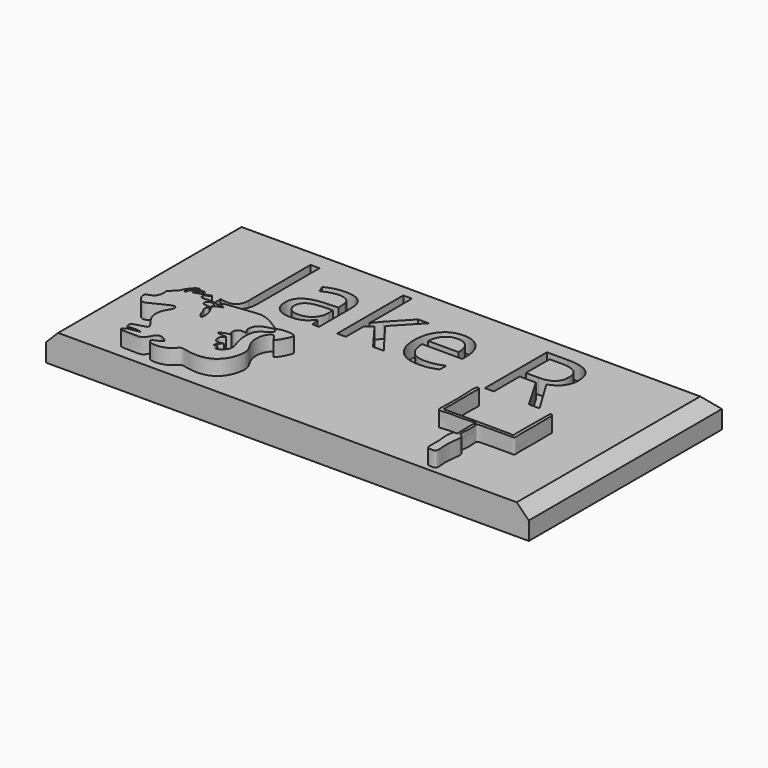
from build123d import *

# Parameters (mm, degrees)
F0_W         = 101.6
F0_H         = 50.8
F1_DEPTH     = 6.35
F2_TEXT_SIZE = 22.889892312
F3_DEPTH     = 3.175
F6_DEPTH     = 3.175
F8_DEPTH     = 3.175
F9_SIZE      = 2.54


# Not quite as in the source:
# - Text() gives the source's letters only with a copy of the font that has no kerning and outlines rounded to 1/6400 em; it was checked with that copy


with BuildPart() as f1:
    # F0 (on Top) → F1 (new body)
    with BuildSketch(Plane.XY):
        with Locations((31.7524990533, -6.3369355765)):
            Rectangle(F0_W, F0_H)
    extrude(amount=F1_DEPTH)

    # F2 (on face) → F3 (cut)
    with BuildSketch(Plane.XY.offset(6.35)):
        with Locations((-1.3590687886, -3.2846634276)):
            Text('Jake R', F2_TEXT_SIZE, font='Open Sans', text_align=(TextAlign.LEFT, TextAlign.BOTTOM))
    extrude(amount=-F3_DEPTH, mode=Mode.SUBTRACT)

    # F5 (on face) → F6 (join)
    with BuildSketch(Plane.XY.offset(6.35)):
        with BuildLine():
            add(Edge.make_bspline(
                [(-9.9473167211, -16.8291665614), (-9.6318161308, -16.6093979481), (-8.0839962394, -16.4614298786), (-7.9211876919, -14.0293243028), (-8.3789792586, -13.9112234461), (-6.3385914042, -12.0992000222), (-6.5202812577, -11.8356315571), (-5.2656681133, -10.0118497624), (-4.5534071308, -9.7378645456), (-4.2294561968, -9.7019648093), (-4.3980035932, -9.988698615), (-5.3176847151, -10.4409761465), (-5.7133396144, -11.440009908), (-5.7601749231, -12.0507048992), (-5.3250122812, -12.0166586319), (-5.5151695466, -11.2267993409), (-4.4172648305, -10.4678783041), (-3.8013369692, -10.2413822662), (-3.1664584015, -9.9795622858), (-2.9351873262, -10.0870364506), (-3.6173853606, -10.4333631624), (-4.4106140277, -10.9661153724), (-4.6578929311, -11.6389382333), (-2.9685088968, -10.872611876), (-1.7672060238, -10.5575074617), (-1.1369119673, -10.3099300849), (-1.3782200505, -10.7224404484), (-2.4536131421, -11.0524062418), (-2.3627095497, -12.0366415406), (-1.1805119076, -11.9653257133), (0.5407672641, -11.8701370936), (0.7217330171, -12.3150559399), (-0.4018086187, -12.270141763), (-0.8940503935, -13.3290837491), (-0.0457538349, -13.7435809238), (1.1398694142, -13.5461403967), (0.7699728306, -14.1837469378), (0.5285162187, -14.8135221399), (0.9767861849, -15.3013890012), (1.2067508203, -16.0261665589), (1.4266113794, -16.8041541097), (1.8335409915, -17.2417675619), (2.2896541555, -17.5865197382), (2.3269041493, -16.1396203305), (2.0902824393, -15.2175440987), (1.6059851597, -14.253562876), (1.3203956773, -13.6380943063), (0.8656034334, -13.378915598), (1.6536734035, -13.0102058821), (2.1442638998, -12.6770885728), (3.3244491956, -12.4108420977), (0.1829963842, -11.4779566095), (6.6402986528, -10.9518911639), (9.2079636257, -10.4311276641), (11.5736832476, -11.238028674), (13.213297199, -12.3934022949), (14.5980573697, -13.1660552716), (12.8123999886, -13.4588177694), (10.931038794, -14.193343875), (10.5901748999, -16.3206207186), (11.8353188414, -17.3818853519), (9.5427126702, -16.7472257612), (9.1994806574, -18.7963337624), (10.2773541237, -19.2600223908), (9.2663295553, -19.1819954863), (6.4967182387, -20.3558888921), (10.5627454218, -20.212945517), (8.8804020018, -20.8702686445), (8.9543814012, -21.9589086267), (9.3820569376, -22.9183607691), (11.461742552, -22.2172179196), (10.2513099098, -22.9519144726), (9.6568200022, -24.2677990338), (11.0083795729, -23.4196006133), (10.6327982369, -25.2961685937), (13.026023199, -23.6602826242), (12.8739516315, -21.9171844349), (11.9206539994, -19.6132841054), (11.888703896, -15.6842303702), (14.1445273132, -14.8208379496), (15.0950637719, -13.723427814), (13.9986766358, -13.2344335713), (15.4668397437, -12.5034113795), (18.2212563844, -12.7012871068), (18.3108018209, -13.7225720098), (16.5749799152, -16.8913138268), (16.2288416461, -15.7403926522), (15.1350726404, -14.4041878251), (13.7535681212, -16.8974024437), (14.1147671991, -19.84446665), (16.050570642, -21.9736001244), (15.017821371, -26.3621646569), (12.1212272086, -28.5743888786), (8.461512688, -28.4908414246), (6.1278841385, -27.6501596981), (5.3764562689, -29.6031983885), (1.4909235529, -30.2657864319), (0.3565580975, -28.7618497283), (2.8961466548, -28.2587909889), (2.5691263976, -27.3781704269), (0.2688195568, -26.2098461929), (-0.3947177356, -29.4901391886), (-2.7696127386, -29.0924765704), (-6.0344947484, -29.3270127365), (-5.0841994026, -27.9874742655), (-0.9992238273, -27.8151791835), (-4.31246706, -27.3511275692), (-5.3953686561, -27.8375676712), (-5.7150155523, -26.1452044672), (-2.5489477256, -25.9565184484), (-2.2697713135, -25.0022003531), (-4.5485511423, -22.8712839697), (-4.5498028259, -19.5890004959), (-2.9945255711, -17.9686708735), (-3.5727775293, -16.8589484433), (-4.9502905393, -17.5416548957), (-7.1849009783, -18.5219981727), (-8.6529993142, -19.4630010319), (-9.8014490724, -18.5674546348), (-10.2273597844, -17.3967143235), (-10.131281799, -16.9573113297), (-9.9473167211, -16.8291665614)],
                knots=[0, 0, 0, 0, 0.0097695183, 0.0203897285, 0.0238601521, 0.0354688695, 0.039997664, 0.0507819177, 0.0575959796, 0.0608781059, 0.0641729785, 0.0717647306, 0.0797164829, 0.0849092257, 0.0884011451, 0.0943720494, 0.1027126611, 0.1092543659, 0.1153066413, 0.1177606055, 0.1236401865, 0.1315312873, 0.1358189897, 0.1449327876, 0.154230184, 0.1590795572, 0.1628959838, 0.1707221829, 0.1766413117, 0.184544845, 0.1943955027, 0.1975978506, 0.2048073857, 0.2118532907, 0.2185124212, 0.225768748, 0.2308501428, 0.2369615184, 0.2427439578, 0.2493573514, 0.2561289767, 0.2620766129, 0.2662295349, 0.2742152744, 0.2821295697, 0.2898618068, 0.296155813, 0.3003614273, 0.3063452978, 0.3130961808, 0.3188786182, 0.3271934004, 0.3430166084, 0.3567002693, 0.3680001725, 0.3791696599, 0.3865269989, 0.3948131693, 0.4056591887, 0.4160381913, 0.4229462806, 0.43190969, 0.4412290025, 0.4473693065, 0.4537572142, 0.463549394, 0.4741787129, 0.4807862267, 0.4884929702, 0.4955649281, 0.5043321668, 0.5110913461, 0.5184393523, 0.5248839746, 0.5319004179, 0.5422339318, 0.5519658524, 0.5640508347, 0.5782099625, 0.5895018851, 0.5972250972, 0.6031507702, 0.6111972809, 0.623402794, 0.6302096828, 0.6432163173, 0.6491419841, 0.6575221581, 0.6683993023, 0.6813711886, 0.693684942, 0.7087916162, 0.7227940756, 0.7371143153, 0.7478848688, 0.7576430214, 0.7720463617, 0.7794693289, 0.7899043628, 0.7956193185, 0.8059813777, 0.8175263091, 0.8289078296, 0.8410683234, 0.848141297, 0.8604198394, 0.8705826242, 0.8785859317, 0.8857443046, 0.8982334613, 0.904106576, 0.9168212254, 0.9302175871, 0.940921851, 0.9474768496, 0.9560227018, 0.968228571, 0.9776739611, 0.9859976486, 0.9943034965, 1, 1, 1, 1], degree=3))
        make_face()
    extrude(amount=F6_DEPTH)

    # F7 (on face) → F8 (join)
    with BuildSketch(Plane.XY.offset(6.35)):
        with BuildLine():
            add(Edge.make_bspline(
                [(53.0794151127, -8.7919523939), (52.9438415025, -9.2051142231), (53.1776297006, -11.9439897237), (53.2050127779, -15.2907789982), (52.9793352998, -18.5582737257), (53.4418642334, -19.0087583892), (55.3997578845, -18.5914936278), (57.9342441051, -18.9281073472), (61.2742233864, -18.5275464238), (60.828305169, -18.9811966693), (60.8228638062, -20.4739650428), (60.9109413715, -21.3694914404), (60.8197313606, -22.7626255839), (61.0119177282, -23.6032983334), (60.2482937033, -23.4526963748), (60.047820144, -23.9403470308), (59.8411835794, -25.3323982811), (60.1781962457, -26.936431579), (60.0570812859, -29.1306944041), (60.1343401179, -30.5688596455), (61.0310529395, -30.5641402756), (62.3128566785, -30.6616639077), (61.8365016143, -28.2560992729), (62.1193893471, -25.5681013821), (62.3666505857, -24.2271226532), (61.839233397, -23.3911528675), (61.2366493739, -23.5177795701), (61.5018586651, -21.8522436689), (61.4782045095, -19.8145870685), (61.3087615539, -18.8257979839), (62.4065889888, -18.8870121633), (63.798857838, -18.7615142216), (67.2812354912, -18.8303957002), (68.3522857442, -18.7696098978), (69.2697765342, -18.9041024014), (69.0577917021, -17.640271928), (69.1425702348, -14.9643128877), (69.1639133332, -12.4086065768), (69.0088470025, -9.5829372311), (69.1637247167, -8.7380763952), (68.8917850841, -8.5720953279), (68.5277067798, -8.4519962735), (68.4161945008, -9.0435779579), (68.4652733474, -9.7271883939), (68.4059716271, -10.7252911504), (68.4948321914, -12.2444604957), (68.4023027569, -13.6434516094), (68.4851701745, -15.1985393585), (68.3192392303, -17.2818707916), (68.5910022656, -18.332774345), (67.9208389747, -18.09788848), (66.507049859, -18.171101472), (63.7606957042, -18.1287370812), (61.4655523281, -18.0595465144), (59.4290351141, -18.093908132), (56.2917532611, -18.1851587794), (54.2753676863, -18.0814603349), (53.643670543, -18.1810522009), (53.7488565588, -17.5482910774), (53.773835433, -14.9337553785), (53.6997778259, -13.1344575722), (53.6632349112, -9.7143668663), (53.8323177199, -8.7819579929), (53.521702629, -8.5943420811), (53.2488041672, -8.5708852592), (53.1212714585, -8.6643947938), (53.0794151127, -8.7919523939)],
                knots=[0, 0, 0, 0, 0.0227787101, 0.0498433835, 0.0732816676, 0.082095887, 0.0999380149, 0.1238921723, 0.1462678359, 0.15293396, 0.1692706257, 0.1830135984, 0.199178935, 0.2099663202, 0.2197374382, 0.2285983817, 0.2443623446, 0.2621234417, 0.2826389743, 0.2974528897, 0.3091558283, 0.3220829767, 0.3413106135, 0.3644340933, 0.3801371783, 0.3923048287, 0.4003624198, 0.4163823595, 0.4368978921, 0.4484670898, 0.4605160148, 0.4774753055, 0.5027035368, 0.517386063, 0.528034396, 0.5412561816, 0.5636840968, 0.5863397129, 0.6090862989, 0.6205994182, 0.6275040303, 0.6347317983, 0.6440517093, 0.6555074627, 0.6690405037, 0.6857989947, 0.7018126602, 0.718928419, 0.7390713784, 0.7510086186, 0.7598295984, 0.7760567127, 0.7988153079, 0.8193839178, 0.8387624662, 0.8631691885, 0.8825477367, 0.8913687155, 0.9004307287, 0.9220228966, 0.9418436548, 0.9667657732, 0.9791188367, 0.9861938708, 0.9929674104, 1, 1, 1, 1], degree=3))
        make_face()
    extrude(amount=F8_DEPTH)

    # F9
    f9_edges = [f1.edges().sort_by_distance(p)[0] for p in [
        (-19.047501, -6.336936, 6.35),
        (31.752499, 19.063064, 6.35),
        (82.552499, -6.336936, 6.35),
    ]]
    chamfer(f9_edges, length=F9_SIZE)


solid = f1.part
